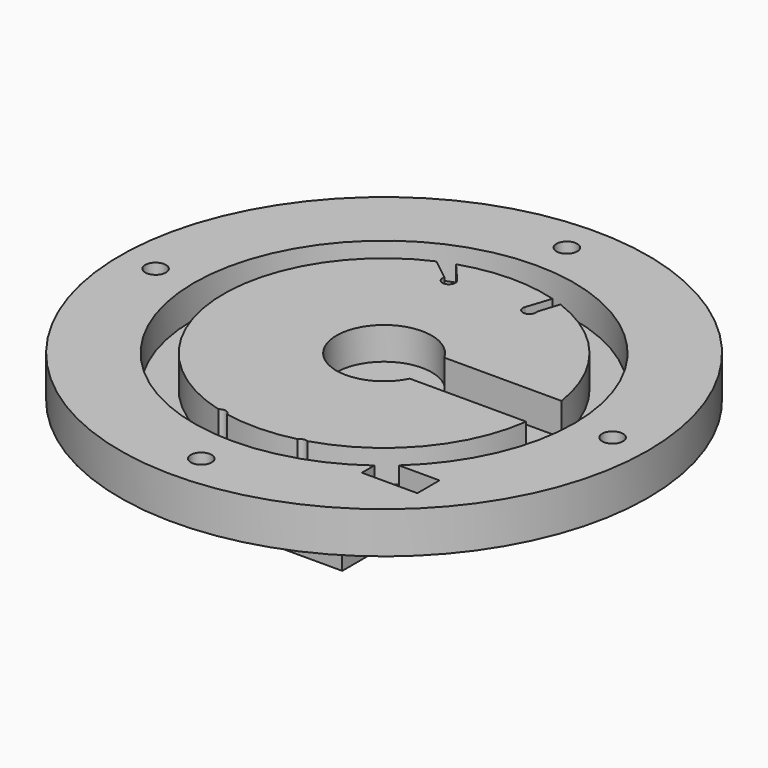
from build123d import *

# Parameters (mm, degrees)
F0_R      = 57.15
F1_DEPTH  = 9
F2_R      = 41.1777557501
F2_R_2    = 34.7361553424
F3_DEPTH  = 7
F5_DEPTH  = 7
F6_W      = 12
F6_H      = 6
F7_DEPTH  = 9
F9_D      = 4.4958
F10_W     = 33
F10_H     = 58
F10_W_2   = 29
F10_H_2   = 54
F11_DEPTH = 14
F13_D     = 2.794
F15_DEPTH = 7


with BuildPart() as f1:
    # F0 (on Top) → F1 (new body)
    with BuildSketch(Plane.XY):
        Circle(F0_R)
    extrude(amount=F1_DEPTH)

    # F2 (on face) → F3 (cut)
    with BuildSketch(Plane.XY.offset(9)):
        Circle(F2_R)
        Circle(F2_R_2, mode=Mode.SUBTRACT)
    extrude(amount=-F3_DEPTH, mode=Mode.SUBTRACT)

    # F4 (on face) → F5 (cut)
    with BuildSketch(Plane.XY.offset(9)):
        with BuildLine():
            ThreePointArc((9.2364512329, -4.5815780759), (10.0382703258, -2.3528743932), (10.3103292403, 0))
            ThreePointArc((10.3103292403, 0), (9.9709085428, 2.6237133751), (8.9749942157, 5.0746790905))
            Line((8.9749942157, 5.0746790905), (8.9749942157, -4.5815780759))
            Line((8.9749942157, -4.5815780759), (9.2364512329, -4.5815780759))
        make_face()
        with BuildLine():
            Line((37.7700850368, 5.0746790905), (34.3634707226, 5.0746790905))
            ThreePointArc((34.3634707226, 5.0746790905), (34.6428588969, 2.544172837), (34.7361553424, 0))
            ThreePointArc((34.7361553424, 0), (34.6602041198, -2.2958088649), (34.4326825895, -4.5815780759))
            Line((34.4326825895, -4.5815780759), (37.7700850368, -4.5815780759))
            Line((37.7700850368, -4.5815780759), (37.7700850368, 5.0746790905))
        make_face()
        with BuildLine():
            Line((8.9749942157, -4.5815780759), (8.9749942157, 5.0746790905))
            ThreePointArc((8.9749942157, 5.0746790905), (-10.3065518942, -0.27906468), (9.2364512329, -4.5815780759))
            Line((9.2364512329, -4.5815780759), (8.9749942157, -4.5815780759))
        make_face()
        with BuildLine():
            ThreePointArc((8.9749942157, 5.0746790905), (9.9709085428, 2.6237133751), (10.3103292403, 0))
            ThreePointArc((10.3103292403, 0), (10.0382703258, -2.3528743932), (9.2364512329, -4.5815780759))
            Line((9.2364512329, -4.5815780759), (34.4326825895, -4.5815780759))
            ThreePointArc((34.4326825895, -4.5815780759), (34.6602041198, -2.2958088649), (34.7361553424, 0))
            ThreePointArc((34.7361553424, 0), (34.6428588969, 2.544172837), (34.3634707226, 5.0746790905))
            Line((34.3634707226, 5.0746790905), (8.9749942157, 5.0746790905))
        make_face()
    extrude(amount=-F5_DEPTH, mode=Mode.SUBTRACT)

    # F6 (on face) → F7 (cut)
    with BuildSketch(Plane(origin=(0, 0, 0), x_dir=(1, 0, 0), z_dir=(0, 0, -1))):
        with Locations((30.4291332662, 33.5408807993)):
            Rectangle(F6_W, F6_H)
    extrude(amount=-F7_DEPTH, mode=Mode.SUBTRACT)

    # F9 (through all)
    with Locations(Plane.XY.offset(9)):
        with Locations((0, 49.4705886591), (-49.4705886591, 0), (0, -49.4705886591), (49.4705886591, 0)):
            Hole(F9_D / 2)

    # F10 (on face) → F11 (join)
    with BuildSketch(Plane(origin=(0, 0, 0), x_dir=(1, 0, 0), z_dir=(0, 0, -1))):
        with Locations((0.185111627, 3.1867184639)):
            Rectangle(F10_W, F10_H)
        with Locations((0.1965364888, 2.9830217808)):
            Rectangle(F10_W_2, F10_H_2, mode=Mode.SUBTRACT)
    extrude(amount=F11_DEPTH)

    # F13 (through all)
    with Locations(Plane(origin=(0, 0, 0), x_dir=(1, 0, 0), z_dir=(0, 0, -1))):
        with Locations((-8.0456975847, 34.5294550061), (9.3866474926, 34.5294550061), (-8.0456975847, -27.6012141258), (9.3866474926, -27.6012141258)):
            Hole(F13_D / 2)

    # F14 (on face) → F15 (cut)
    with BuildSketch(Plane.XY.offset(9)):
        with BuildLine():
            Line((-14.0573482538, 31.7646257344), (-9.3722739345, 28.0391686762))
            ThreePointArc((-9.3722739345, 28.0391686762), (-8.3136402911, 28.9722778391), (-6.9816011946, 28.5063703953))
            Line((-6.9816011946, 28.5063703953), (-10.8128362283, 33.0103477817))
            ThreePointArc((-10.8128362283, 33.0103477817), (-12.4506817042, 32.4280898771), (-14.0573482538, 31.7646257344))
        make_face()
        with BuildLine():
            ThreePointArc((12.1452810093, 32.5437034951), (10.9819164525, 32.9544837466), (9.804697926, 33.3236910704))
            Line((9.804697926, 33.3236910704), (8.0600711429, 28.0391686762))
            ThreePointArc((8.0600711429, 28.0391686762), (9.3866474926, 28.9982141258), (10.7132238424, 28.0391686762))
            Line((10.7132238424, 28.0391686762), (12.1452810093, 32.5437034951))
        make_face()
    extrude(amount=-F15_DEPTH, mode=Mode.SUBTRACT)


solid = f1.part
